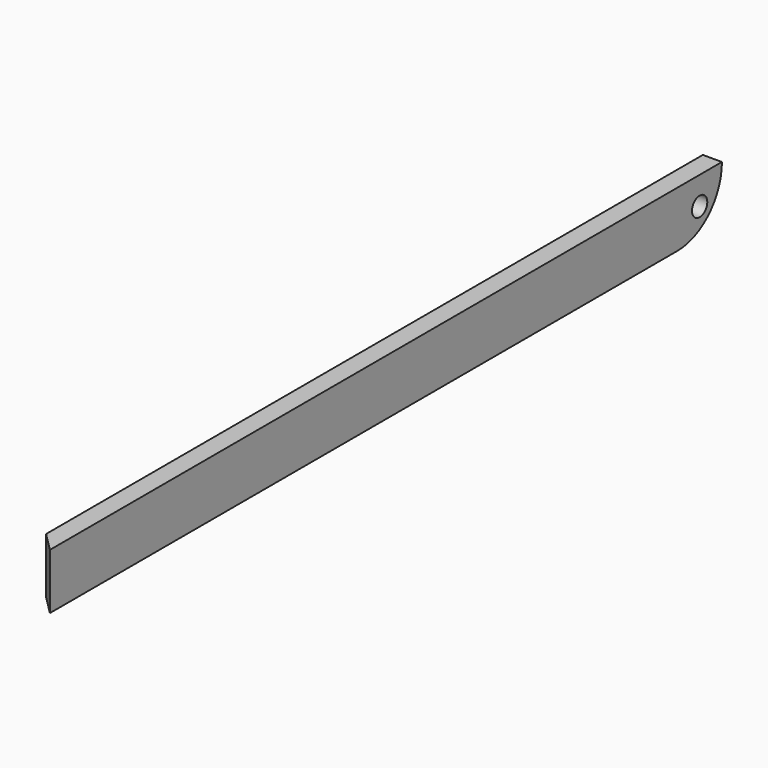
from build123d import *

# Parameters (mm, degrees)
F0_W     = 838.2
F0_H     = 55.5625
F1_DEPTH = 19.05
F2_R     = 55.56249
F4_DEPTH = 55.5635
F5_R     = 9.525
F6_DEPTH = 25.4


# Not quite as in the source:
# - a fillet or chamfer is up to 0.001 mm smaller than in the source, because OpenCascade refuses the exact size


with BuildPart() as f1:
    # F0 (on Right) → F1 (new body)
    with BuildSketch(Plane.YZ):
        Rectangle(F0_W, F0_H)
    extrude(amount=F1_DEPTH)

    # F2 (radius 55.5625 in the source; OpenCascade refuses exactly that, so slightly less here)
    f2_edges = [f1.edges().sort_by_distance(p)[0] for p in [
        (9.525, 419.1, -27.78125),
    ]]
    fillet(f2_edges, radius=F2_R)

    # F3 (on face) → F4 (cut, through all)
    with BuildSketch(Plane.XY.offset(27.78125)):
        Polygon((0, -419.1), (19.05, -419.1), (0, -400.05), align=None)
    extrude(amount=-F4_DEPTH, mode=Mode.SUBTRACT)

    # F5 (on face) → F6 (cut)
    with BuildSketch(Plane.YZ.offset(19.05)):
        with Locations((391.31875, 0)):
            Circle(F5_R)
    extrude(amount=-F6_DEPTH, mode=Mode.SUBTRACT)


solid = f1.part
